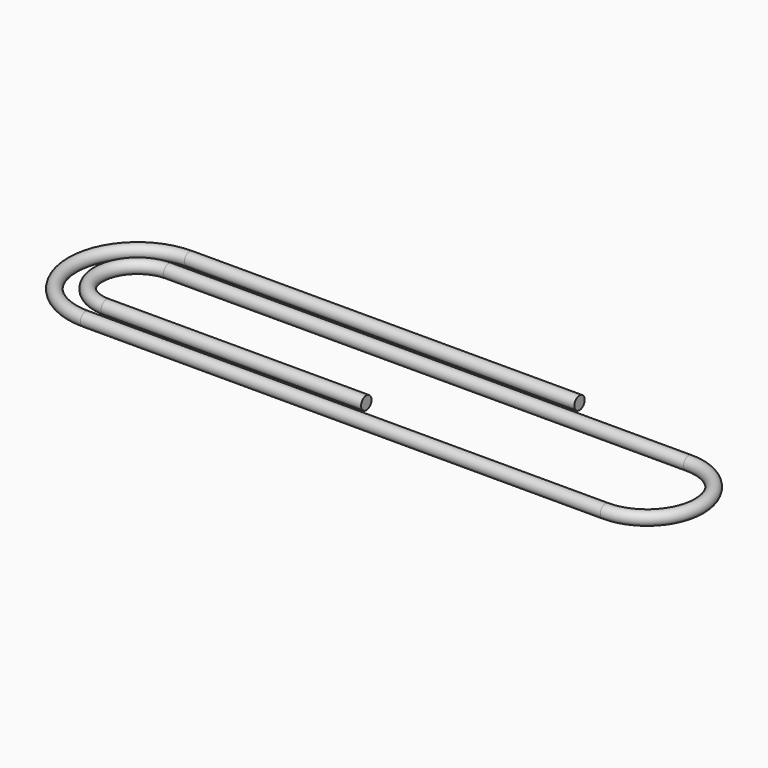
from build123d import *

# Parameters (mm, degrees)
F1_R = 0.635


with BuildPart() as f2:
    # F2: sweep along a path in F0
    with BuildLine(Plane.XY) as f2_path:
        Line((12.7, 10.16), (-25.4, 10.16))
        ThreePointArc((-25.4, 10.16), (-31.75, 3.81), (-25.4, -2.54))
        Line((-25.4, -2.54), (25.4, -2.54))
        ThreePointArc((25.4, -2.54), (30.48, 2.54), (25.4, 7.62))
        Line((25.4, 7.62), (-25.4, 7.62))
        ThreePointArc((-25.4, 7.62), (-29.21, 3.81), (-25.4, 0))
        Line((-25.4, 0), (0, 0))
    # F1 (on Right) → F2 (sweep)
    with BuildSketch(Plane.YZ):
        Circle(F1_R)
    sweep(path=f2_path.line)


solid = f2.part
